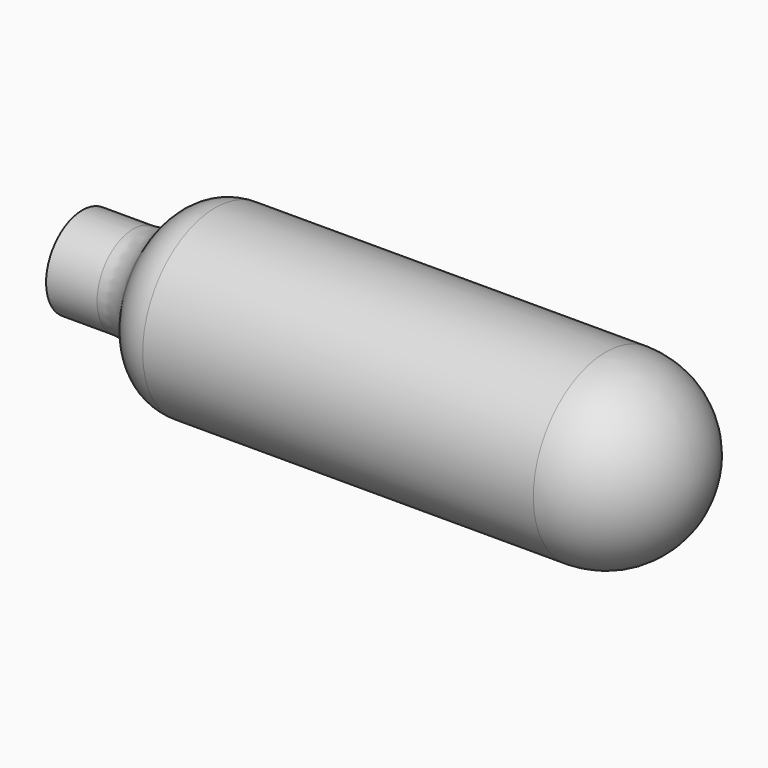
from build123d import *

# Parameters (mm, degrees)
F2_R = 9.525
F4_R = 5.08


# Not quite as in the source:
# - a fillet or chamfer that OpenCascade refuses, or shapes differently, is made with other operations: its cross-section is extruded or revolved along the edge and cut away or added


with BuildPart() as f1:
    # F0 (on Front) → F1 (revolve)
    with BuildSketch(Plane.XZ):
        Polygon((0, 4.7625), (0, 0), (64.516, 0), (64.516, 9.525), (8.89, 9.525), (8.89, 4.7625), align=None)
    revolve(axis=Axis((32.258, 0, 0), (-1, 0, 0)))

    # F2
    f2_edges = [f1.edges().sort_by_distance(p)[0] for p in [
        (64.516, 0, -9.525),
    ]]
    fillet(f2_edges, radius=F2_R)

    # F3: fillet of radius 5.08 on 1 edges, made by hand

    # F3_s1 → F3_t2 (revolve, cut)
    with BuildSketch(Plane.XZ):
        with BuildLine():
            ThreePointArc((13.9600684167, 9.525), (10.4820301765, 8.1476544532), (8.89, 4.7625))
            Line((8.89, 4.7625), (8.89, 9.525))
            Line((8.89, 9.525), (13.9600684167, 9.525))
        make_face()
    revolve(axis=Axis((8.89, 0, 0), (-1, 0, 0)), mode=Mode.SUBTRACT)

    # F4
    f4_edges = [f1.edges().sort_by_distance(p)[0] for p in [
        (8.89, 0, -4.7625),
    ]]
    fillet(f4_edges, radius=F4_R)


solid = f1.part
